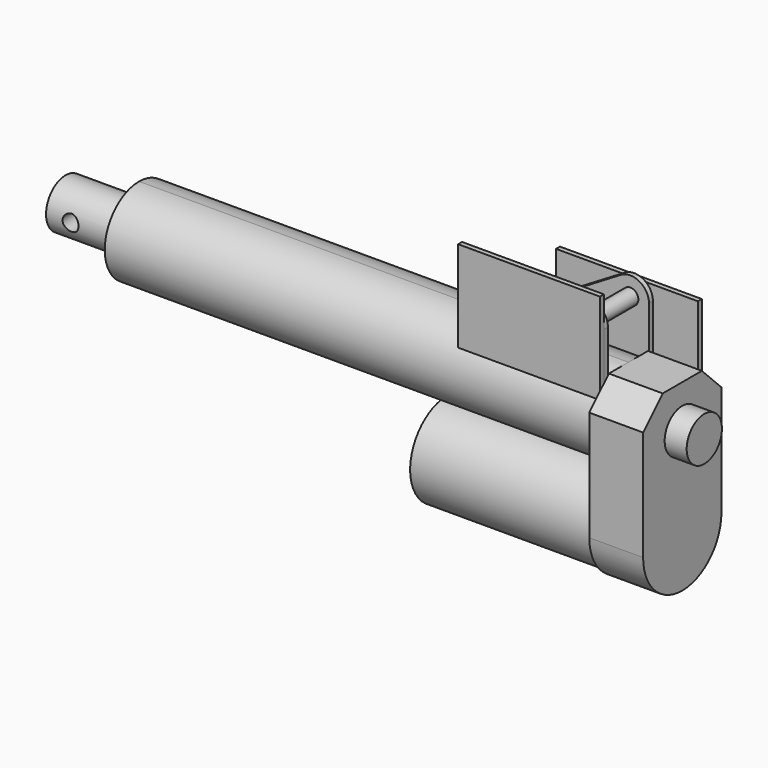
from build123d import *

# Parameters (mm, degrees)
F2_R      = 19
F2_R_2    = 10
F2_R_3    = 9
F3_DEPTH  = 22
F4_DEPTH  = 74
F5_DEPTH  = 200
F6_DEPTH  = 31
F7_R      = 10
F8_DEPTH  = 230
F9_R      = 3.25
F10_DEPTH = 10
F11_R     = 3.25
F12_DEPTH = 10
F13_R     = 3.25
F13_W     = 58
F13_H     = 3
F14_DEPTH = 12.5
F15_DEPTH = 10.5
F16_DEPTH = 12.5
F18_DEPTH = 58
F20_DEPTH = 58
F21_R     = 4.1
F22_DEPTH = 5


with BuildPart() as f3:
    # F2 (on Right) → F3 (new body)
    with BuildSketch(Plane.YZ):
        with BuildLine():
            Line((-10, 17.5), (-20, 7.5))
            Line((-20, 7.5), (-20, -37.5))
            ThreePointArc((-20, -37.5), (0, -57.5), (20, -37.5))
            Line((20, -37.5), (20, 7.5))
            Line((20, 7.5), (10, 17.5))
            Line((10, 17.5), (0, 17.5))
            Line((0, 17.5), (-10, 17.5))
        make_face()
        with Locations((0, -37.5)):
            Circle(F2_R, mode=Mode.SUBTRACT)
        with BuildLine():
            ThreePointArc((17.5, 0), (-12.3743686708, -12.3743686708), (0, 17.5))
            ThreePointArc((0, 17.5), (12.3743686708, 12.3743686708), (17.5, 0))
        make_face(mode=Mode.SUBTRACT)
        with Locations((0, -37.5)):
            Circle(F2_R)
        with BuildLine():
            ThreePointArc((17.5, 0), (12.3743686708, 12.3743686708), (0, 17.5))
            ThreePointArc((0, 17.5), (-12.3743686708, -12.3743686708), (17.5, 0))
        make_face()
        Circle(F2_R_2, mode=Mode.SUBTRACT)
        Circle(F2_R_2)
        Circle(F2_R_3, mode=Mode.SUBTRACT)
        Circle(F2_R_3)
    extrude(amount=F3_DEPTH)

    # F2 (on Right) → F4 (join)
    with BuildSketch(Plane.YZ):
        with Locations((0, -37.5)):
            Circle(F2_R)
    extrude(amount=-F4_DEPTH)

    # F2 (on Right) → F5 (join)
    with BuildSketch(Plane.YZ):
        with BuildLine():
            ThreePointArc((17.5, 0), (12.3743686708, 12.3743686708), (0, 17.5))
            ThreePointArc((0, 17.5), (-12.3743686708, -12.3743686708), (17.5, 0))
        make_face()
        Circle(F2_R_2, mode=Mode.SUBTRACT)
    extrude(amount=-F5_DEPTH)

    # F2 (on Right) → F6 (join)
    with BuildSketch(Plane.YZ):
        Circle(F2_R_3)
    extrude(amount=F6_DEPTH)

    # F11 (on Front) → F12 (cut, symmetric)
    with BuildSketch(Plane.XZ):
        with Locations((40, 0)):
            Circle(F11_R)
    extrude(amount=F12_DEPTH, both=True, mode=Mode.SUBTRACT)


with BuildPart() as f8:
    # F7 (on Right) → F8 (new body)
    with BuildSketch(Plane.YZ):
        Circle(F7_R)
    extrude(amount=-F8_DEPTH)

    # F9 (on Front) → F10 (cut, symmetric)
    with BuildSketch(Plane.XZ):
        with Locations((-220, 0)):
            Circle(F9_R)
    extrude(amount=F10_DEPTH, both=True, mode=Mode.SUBTRACT)


with BuildPart() as f14:
    # F13 (on Front) → F14 (new body, symmetric)
    with BuildSketch(Plane.XZ):
        with BuildLine():
            Line((-58, 0), (0, 0))
            Line((0, 0), (0, 34.4))
            ThreePointArc((0, 34.4), (-3.8566941985, 41.0142015147), (-11.5125425465, 40.9155207637))
            Line((-11.5125425465, 40.9155207637), (-58, 13))
            Line((-58, 13), (-58, 0))
        make_face()
        with Locations((-7.6, 34.4)):
            Circle(F13_R, mode=Mode.SUBTRACT)
        with Locations((-29, -1.5)):
            Rectangle(F13_W, F13_H)
    extrude(amount=F14_DEPTH, both=True)

    # F13 (on Front) → F15 (cut, symmetric)
    with BuildSketch(Plane.XZ):
        with BuildLine():
            Line((-58, 0), (0, 0))
            Line((0, 0), (0, 34.4))
            ThreePointArc((0, 34.4), (-3.8566941985, 41.0142015147), (-11.5125425465, 40.9155207637))
            Line((-11.5125425465, 40.9155207637), (-58, 13))
            Line((-58, 13), (-58, 0))
        make_face()
        with Locations((-7.6, 34.4)):
            Circle(F13_R, mode=Mode.SUBTRACT)
    extrude(amount=F15_DEPTH, both=True, mode=Mode.SUBTRACT)

    # F13 (on Front) → F16 (join, symmetric)
    with BuildSketch(Plane.XZ):
        with Locations((-7.6, 34.4)):
            Circle(F13_R)
    extrude(amount=F16_DEPTH, both=True)

    # F21 (on face) → F22 (cut)
    with BuildSketch(Plane(origin=(0, 0, -3), x_dir=(1, 0, 0), z_dir=(0, 0, -1))):
        with Locations((-45.9, 0)):
            Circle(F21_R)
        with BuildLine():
            Line((0, 4.5), (-9.5, 4.5))
            ThreePointArc((-9.5, 4.5), (-14, 0), (-9.5, -4.5))
            Line((-9.5, -4.5), (0, -4.5))
            Line((0, -4.5), (0, 4.5))
        make_face()
    extrude(amount=-F22_DEPTH, mode=Mode.SUBTRACT)


with BuildPart() as f18:
    # F17 (on face) → F18 (new body)
    with BuildSketch(Plane.YZ):
        Polygon((-14.5, -5), (20.5, -5), (20.5, -3), (-12.5, -3), (-12.5, 47), (-14.5, 47), align=None)
    extrude(amount=-F18_DEPTH)


with BuildPart() as f20:
    # F19 (on face) → F20 (new body)
    with BuildSketch(Plane.YZ):
        Polygon((12.5, -3), (-12.5, -3), (-12.5, -5), (37.5, -5), (37.5, 25), (35.5, 25), (35.5, -3), align=None)
    extrude(amount=-F20_DEPTH)


solid = Compound([f3.part, f8.part, f14.part, f18.part, f20.part])
